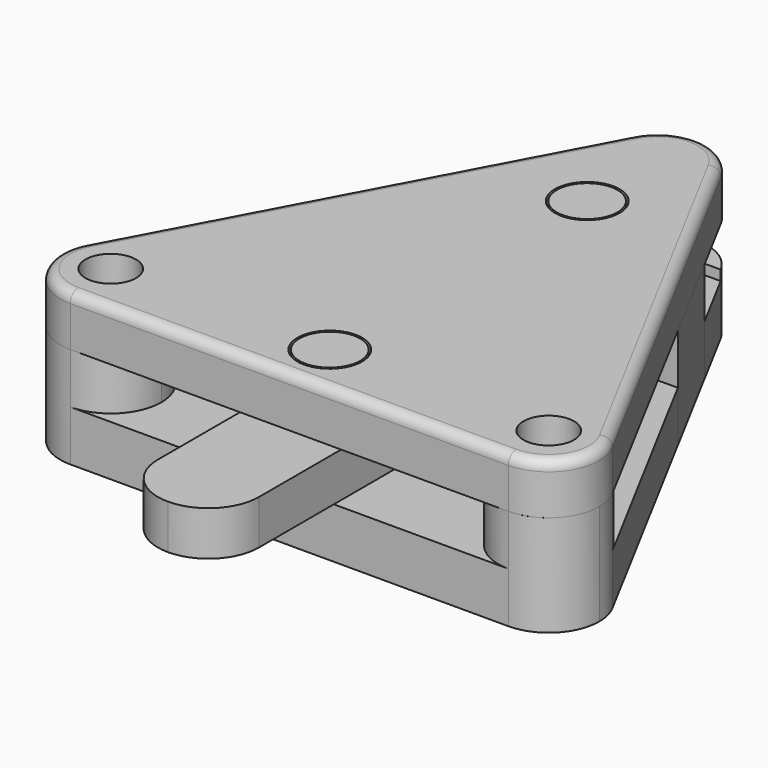
from build123d import *

# Parameters (mm, degrees)
F0_R      = 3.81
F1_DEPTH  = 6.35
F0_R_2    = 3.175
F2_DEPTH  = 12.7
F3_DEPTH  = 19.05
F4_DEPTH  = 7.62
F7_START  = 6.35
F6_R      = 3.175
F6_R_2    = 4.064
F7_DEPTH  = 6.35
F8_R      = 1.27
F10_START = 0.635
F9_R      = 4.318
F10_DEPTH = 5.588


# Not quite as in the source:
# - a feature names something its author has since deleted; it is built from what else it names


with BuildPart() as f1:
    # F0 (on Top) → F1 (new body)
    with BuildSketch(Plane.XY):
        with BuildLine():
            Line((-27.4988556353, -35.5915231094), (27.4988556353, -35.5915231094))
            ThreePointArc((27.4988556353, -35.5915231094), (22.0513543675, -25.9785137718), (33.0973587859, -26.2449813572))
            Line((33.0973587859, -26.2449813572), (16.4745760518, 4.811719736))
            Line((16.4745760518, 4.811719736), (-16.4745760518, 4.811719736))
            Line((-16.4745760518, 4.811719736), (-33.0973587859, -26.2449813572))
            ThreePointArc((-33.0973587859, -26.2449813572), (-25.954186578, -23.0822619927), (-21.1488556353, -29.2415231094))
            ThreePointArc((-21.1488556353, -29.2415231094), (-23.0087275748, -33.7316511699), (-27.4988556353, -35.5915231094))
        make_face()
        with Locations((0, -29.2415231094)):
            Circle(F0_R, mode=Mode.SUBTRACT)
    extrude(amount=F1_DEPTH)



with BuildPart() as f1b:
    # F0 (on Top) → F1, piece 2 (new body)
    with BuildSketch(Plane.XY):
        Polygon((-9.6770304886, 17.511719736), (9.6770304886, 17.511719736), (5.5985031506, 25.131719736), (-5.5985031506, 25.131719736), align=None)
    extrude(amount=F1_DEPTH)


with BuildPart() as f1_1:
    add(f1.part)

    add(f1b.part)  # F2 merges F1b
    # F0 (on Top) → F2 (join)
    with BuildSketch(Plane.XY):
        Polygon((-16.4745760518, 4.811719736), (16.4745760518, 4.811719736), (9.6770304886, 17.511719736), (-9.6770304886, 17.511719736), align=None)
        with Locations((0, 11.161719736)):
            Circle(F0_R, mode=Mode.SUBTRACT)
        with BuildLine():
            ThreePointArc((-33.0973587859, -26.2449813572), (-32.9463569031, -32.5045324469), (-27.4988556353, -35.5915231094))
            ThreePointArc((-27.4988556353, -35.5915231094), (-23.0087275748, -33.7316511699), (-21.1488556353, -29.2415231094))
            ThreePointArc((-21.1488556353, -29.2415231094), (-25.954186578, -23.0822619927), (-33.0973587859, -26.2449813572))
        make_face()
        with Locations((-27.4988556353, -29.2415231094)):
            Circle(F0_R_2, mode=Mode.SUBTRACT)
        with BuildLine():
            ThreePointArc((33.0973587859, -26.2449813572), (22.0513543675, -25.9785137718), (27.4988556353, -35.5915231094))
            ThreePointArc((27.4988556353, -35.5915231094), (31.9889836958, -33.7316511699), (33.8488556353, -29.2415231094))
            ThreePointArc((33.8488556353, -29.2415231094), (33.658116752, -27.696854052), (33.0973587859, -26.2449813572))
        make_face()
        with Locations((27.4988556353, -29.2415231094)):
            Circle(F0_R_2, mode=Mode.SUBTRACT)
    extrude(amount=F2_DEPTH)

    # F0 (on Top) → F3 (join)
    with BuildSketch(Plane.XY):
        with Locations((0, -29.2415231094)):
            Circle(F0_R)
        with Locations((0, 11.161719736)):
            Circle(F0_R)
    extrude(amount=F3_DEPTH)

    # F0 (on Top) → F4 (join)
    with BuildSketch(Plane.XY):
        with BuildLine():
            Line((-5.5985031506, 25.131719736), (5.5985031506, 25.131719736))
            ThreePointArc((5.5985031506, 25.131719736), (0, 28.4851779838), (-5.5985031506, 25.131719736))
        make_face()
    extrude(amount=F4_DEPTH)


with BuildPart() as f7:
    # F6 (on offset) → F7 (new body)
    with BuildSketch(Plane.XY.offset(6.35).offset(F7_START)):
        with BuildLine():
            ThreePointArc((-33.1054605215, -26.2434523784), (-32.9535893922, -32.5024634142), (-27.5063946063, -35.5889424682))
            Line((-27.5063946063, -35.5889424682), (27.4986321348, -35.5889424682))
            ThreePointArc((27.4986321348, -35.5889424682), (32.9456677616, -32.5027290543), (33.0979901862, -26.2439984934))
            Line((33.0979901862, -26.2439984934), (5.5987015339, 25.1687706999))
            ThreePointArc((5.5987015339, 25.1687706999), (-0.0003468463, 28.5238267175), (-5.5997224327, 25.1693168148))
            Line((-5.5997224327, 25.1693168148), (-33.1054605215, -26.2434523784))
        make_face()
        with Locations((-27.5063946063, -29.2389424682)):
            Circle(F6_R, mode=Mode.SUBTRACT)
        with Locations((0, -29.2357727885)):
            Circle(F6_R_2, mode=Mode.SUBTRACT)
        with Locations((27.4986321348, -29.2389424682)):
            Circle(F6_R, mode=Mode.SUBTRACT)
        with Locations((0, 11.1793484539)):
            Circle(F6_R_2, mode=Mode.SUBTRACT)
    extrude(amount=F7_DEPTH)

    # F8
    f8_edges = [f7.edges().sort_by_distance(p)[0] for p in [
        (-0.003881, -35.588942, 19.05),
        (-19.352591, -0.537068, 19.05),
        (-32.953589, -32.502463, 19.05),
        (32.945668, -32.502729, 19.05),
        (19.348346, -0.537614, 19.05),
        (-0.000347, 28.523827, 19.05),
    ]]
    fillet(f8_edges, radius=F8_R)


with BuildPart() as f10:
    # F9 (on offset) → F10 (new body)
    with BuildSketch(Plane.XY.offset(6.35).offset(F10_START)):
        with BuildLine():
            Line((6.35, -8.0273897686), (-6.35, -8.0273897686))
            Line((-6.35, -8.0273897686), (-6.35, -48.2915231094))
            ThreePointArc((-6.35, -48.2915231094), (-4.4901280605, -52.7816511699), (0, -54.6415231094))
            ThreePointArc((0, -54.6415231094), (4.4901280605, -52.7816511699), (6.35, -48.2915231094))
            Line((6.35, -48.2915231094), (6.35, -8.0273897686))
        make_face()
        with Locations((0, -29.2415231094)):
            Circle(F9_R, mode=Mode.SUBTRACT)
        with BuildLine():
            ThreePointArc((-5.588, 1.5509696046), (-8.3397511172, -2.853894355), (-7.8815962098, -8.0273897686))
            Line((-7.8815962098, -8.0273897686), (-6.35, -8.0273897686))
            Line((-6.35, -8.0273897686), (6.35, -8.0273897686))
            Line((6.35, -8.0273897686), (7.1399843125, -8.0273897686))
            Line((7.1399843125, -8.0273897686), (12.6776003079, -8.0273897686))
            Line((12.6776003079, -8.0273897686), (12.6776003079, -1.665280264))
            ThreePointArc((12.6776003079, -1.665280264), (11.1976135326, 1.918893948), (7.62, 3.4146703512))
            Line((7.62, 3.4146703512), (7.1119572316, 2.5348132347))
            Line((7.1119572316, 2.5348132347), (6.604, 3.414719736))
            Line((6.604, 3.414719736), (5.588, 3.414719736))
            Line((5.588, 3.414719736), (5.08, 2.5348379257))
            Line((5.08, 2.5348379257), (4.572, 3.414719736))
            Line((4.572, 3.414719736), (3.556, 3.414719736))
            Line((3.556, 3.414719736), (3.048, 2.5348379257))
            Line((3.048, 2.5348379257), (2.54, 3.414719736))
            Line((2.54, 3.414719736), (1.524, 3.414719736))
            Line((1.524, 3.414719736), (1.016, 2.5348379257))
            Line((1.016, 2.5348379257), (0.508, 3.414719736))
            Line((0.508, 3.414719736), (0, 3.414719736))
            Line((0, 3.414719736), (-0.508, 3.414719736))
            Line((-0.508, 3.414719736), (-0.9487344679, 2.4992913505))
            Line((-0.9487344679, 2.4992913505), (-1.524, 3.3367431805))
            ThreePointArc((-1.524, 3.3367431805), (-2.0353121388, 3.248589027), (-2.54, 3.1281671814))
            Line((-2.54, 3.1281671814), (-2.7671357963, 2.1378817023))
            Line((-2.7671357963, 2.1378817023), (-3.556, 2.7781545099))
            ThreePointArc((-3.556, 2.7781545099), (-4.0729321621, 2.5395770195), (-4.572, 2.2655891141))
            Line((-4.572, 2.2655891141), (-4.617414163, 1.250604605))
            Line((-4.617414163, 1.250604605), (-5.588, 1.5509696046))
        make_face()
    extrude(amount=F10_DEPTH)


solid = Compound([f1_1.part, f7.part, f10.part])
